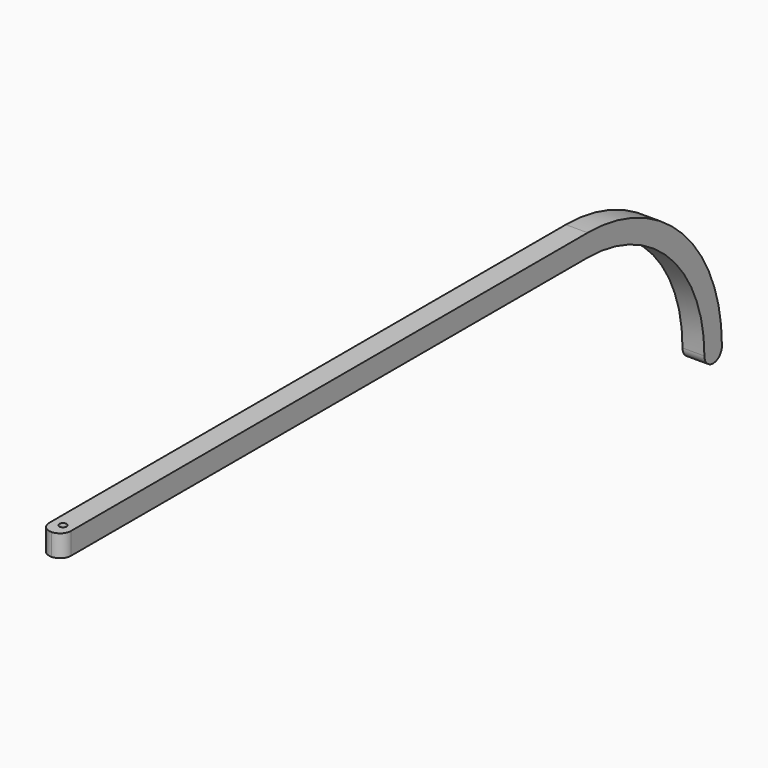
from build123d import *

# Parameters (mm, degrees)
F1_DEPTH = 3
F3_D     = 1
F4_R     = 1.49999


# Not quite as in the source:
# - a fillet or chamfer is up to 0.001 mm smaller than in the source, because OpenCascade refuses the exact size
# - ends of sketch curves that miss each other by under 0.0002 mm in the source are joined


with BuildPart() as f1:
    # F0 (on Right) → F1 (new body)
    with BuildSketch(Plane.YZ):
        with BuildLine():
            Line((-45, 3), (-45, 0))
            Line((-45, 0), (45, 0))
            ThreePointArc((45, 0), (59.1421356237, -5.8578643763), (65, -20))
            ThreePointArc((65, -20), (66.5000000156, -21.499999553), (68, -19.999999553))
            ThreePointArc((68, -19.999999553), (61.2634559673, -3.7365440327), (45, 3))
            Line((45, 3), (-45, 3))
        make_face()
    extrude(amount=F1_DEPTH)

    # F3 (through all)
    with Locations(Plane(origin=(0, 0, 0), x_dir=(1, 0, 0), z_dir=(0, 0, -1))):
        with Locations((1.5, 43)):
            Hole(F3_D / 2)

    # F4 (radius 1.5 in the source; OpenCascade refuses exactly that, so slightly less here)
    f4_edges = [f1.edges().sort_by_distance(p)[0] for p in [
        (3, -45, 1.5),
        (0, -45, 1.5),
    ]]
    fillet(f4_edges, radius=F4_R)


solid = f1.part
